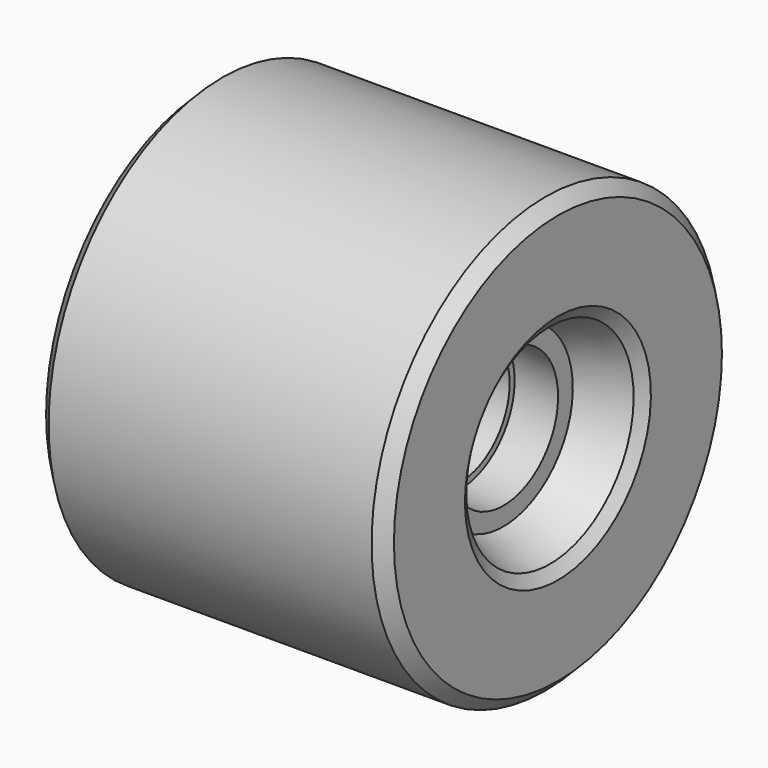
from build123d import *


# Not quite as in the source:
# - a fillet or chamfer that OpenCascade refuses, or shapes differently, is made with other operations: its cross-section is extruded or revolved along the edge and cut away or added


with BuildPart() as f1:
    # F0 (on Front) → F1 (revolve)
    with BuildSketch(Plane.XZ):
        Polygon((-15.7733729929, 11), (-8.7733729929, 11), (-8.7733729929, 13.9589581495), (0, 17.3333312895), (0, 35), (-56, 35), (-56, 24.5486367494), (-28.7733729929, 12.9255643114), (-28.7733729929, 11), (-21.7733729929, 11), (-21.7733729929, 10), (-15.7733729929, 10), align=None)
    revolve(axis=Axis((-19.2243028432, 0, 0), (-1, 0, 0)))

    # F2: chamfer of 2 on 3 edges, made by hand

    # F2_s1 → F2_t2 (revolve, cut)
    with BuildSketch(Plane.XZ):
        Polygon((0, 33), (-2, 35), (0, 35), align=None)
    revolve(axis=Axis((0, 0, 0), (-1, 0, 0)), mode=Mode.SUBTRACT)

    # F2_s3 → F2_t4 (revolve, cut)
    with BuildSketch(Plane.XZ):
        Polygon((-54, 35), (-56, 33), (-56, 35), align=None)
    revolve(axis=Axis((-56, 0, 0), (-1, 0, 0)), mode=Mode.SUBTRACT)

    # F2_s5 → F2_t6 (revolve, cut)
    with BuildSketch(Plane.XZ):
        Polygon((-1.2820420431, 16.840238355), (0, 18.706929645), (0, 17.3333312895), align=None)
    revolve(axis=Axis((0, 0, 0), (-1, 0, 0)), mode=Mode.SUBTRACT)


solid = f1.part
